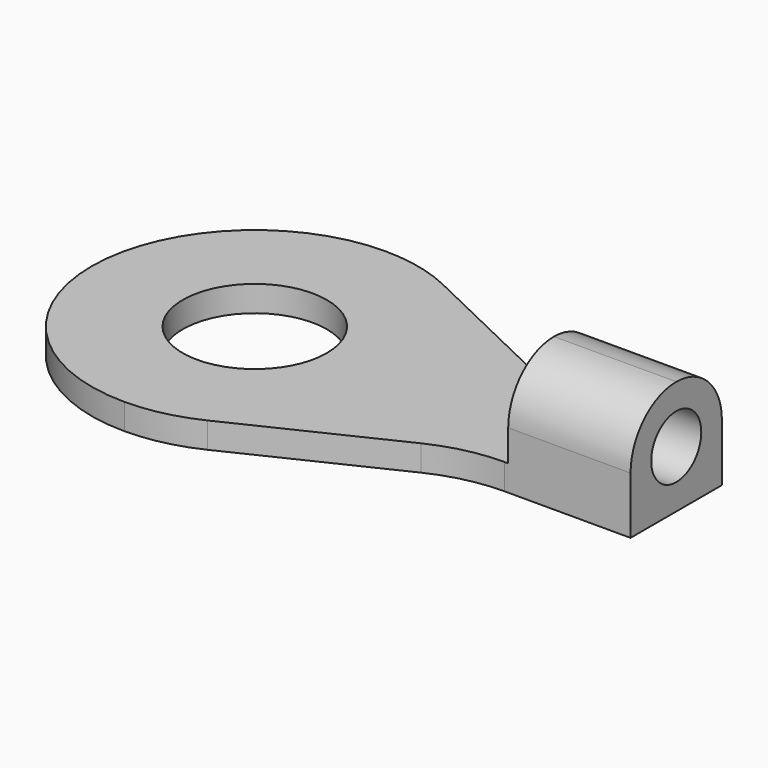
from build123d import *

# Parameters (mm, degrees)
F0_R     = 2.65
F1_DEPTH = 0.95
F2_W     = 4.5
F2_H     = 4.2
F3_DEPTH = 3.25
F4_R     = 2.09999
F5_R     = 1.15
F6_DEPTH = 25


# Not quite as in the source:
# - a fillet or chamfer is up to 0.001 mm smaller than in the source, because OpenCascade refuses the exact size


with BuildPart() as f1:
    # F0 (on Top) → F1 (new body)
    with BuildSketch(Plane.XY):
        with BuildLine():
            Line((16.8637172922, 3.9), (21.5, 3.9))
            Line((21.5, 3.9), (21.5, 8.1))
            Line((21.5, 8.1), (16.8637172922, 8.1))
            ThreePointArc((16.8637172922, 8.1), (15.5339156309, 8.2492199202), (14.2702582689, 8.6894574861))
            Line((14.2702582689, 8.6894574861), (8.5934590232, 11.4105425139))
            ThreePointArc((8.5934590232, 11.4105425139), (7.3298016613, 11.8507800798), (6, 12))
            ThreePointArc((6, 12), (1.7573593129, 10.2426406871), (0, 6))
            ThreePointArc((0, 6), (1.7573593129, 1.7573593129), (6, 0))
            ThreePointArc((6, 0), (7.3298016613, 0.1492199202), (8.5934590232, 0.5894574861))
            Line((8.5934590232, 0.5894574861), (14.2702582689, 3.3105425139))
            ThreePointArc((14.2702582689, 3.3105425139), (15.5339156309, 3.7507800798), (16.8637172922, 3.9))
        make_face()
        with Locations((6, 6)):
            Circle(F0_R, mode=Mode.SUBTRACT)
    extrude(amount=F1_DEPTH)

    # F2 (on face) → F3 (join)
    with BuildSketch(Plane.XY.offset(0.95)):
        with Locations((19.25, 6)):
            Rectangle(F2_W, F2_H)
    extrude(amount=F3_DEPTH)

    # F4 (radius 2.1 in the source; OpenCascade refuses exactly that, so slightly less here)
    f4_edges = [f1.edges().sort_by_distance(p)[0] for p in [
        (19.25, 8.1, 4.2),
        (19.25, 3.9, 4.2),
    ]]
    fillet(f4_edges, radius=F4_R)

    # F5 (on face) → F6 (cut)
    with BuildSketch(Plane.YZ.offset(21.5)):
        with Locations((6, 2.1)):
            Circle(F5_R)
    extrude(amount=-F6_DEPTH, mode=Mode.SUBTRACT)


solid = f1.part
